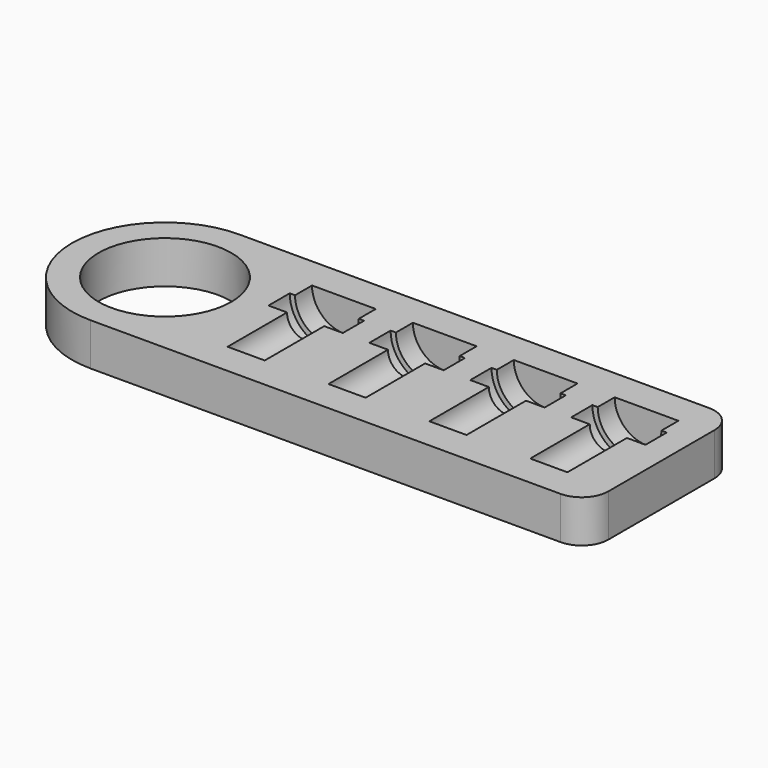
from build123d import *

# Parameters (mm, degrees)
F0_R         = 12.5
F1_DEPTH     = 8
F7_TEXT_SIZE = 5.5555555556
F8_DEPTH     = 1


# Not quite as in the source:
# - Text() gives the source's letters only with a copy of the font that has no kerning and outlines rounded to 1/6400 em; it was checked with that copy


with BuildPart() as f1:
    # F0 (on Top) → F1 (new body)
    with BuildSketch(Plane.XY):
        with BuildLine():
            ThreePointArc((0, 17.5), (5.1256313292, 5.1256313292), (17.5, 0))
            Line((17.5, 0), (106, 0))
            ThreePointArc((106, 0), (109.5355339059, 1.4644660941), (111, 5))
            Line((111, 5), (111, 30))
            ThreePointArc((111, 30), (109.5355339059, 33.5355339059), (106, 35))
            Line((106, 35), (17.5, 35))
            ThreePointArc((17.5, 35), (5.1256313292, 29.8743686708), (0, 17.5))
        make_face()
        with Locations((17.5, 17.5)):
            Circle(F0_R, mode=Mode.SUBTRACT)
    extrude(amount=F1_DEPTH)

    # F2 (on face) → F3 (revolve, cut)
    with BuildSketch(Plane.XY.offset(8)):
        Polygon((42, 20), (42, 6), (45.5, 6), (45.5, 20), (49, 20), (49, 25), (48, 25), (48, 29), (42, 29), (42, 25), align=None)
    revolve(axis=Axis((42, 22.5, 8), (0, 1, 0)), mode=Mode.SUBTRACT)

    # F2 (on face) → F4 (revolve, cut)
    with BuildSketch(Plane.XY.offset(8)):
        Polygon((61, 20), (61, 6), (64.5, 6), (64.5, 20), (68, 20), (68, 25), (67, 25), (67, 29), (61, 29), (61, 25), align=None)
    revolve(axis=Axis((61, 22.5, 8), (0, 1, 0)), mode=Mode.SUBTRACT)

    # F2 (on face) → F5 (revolve, cut)
    with BuildSketch(Plane.XY.offset(8)):
        Polygon((80, 20), (80, 6), (83.5, 6), (83.5, 20), (87, 20), (87, 25), (86, 25), (86, 29), (80, 29), (80, 25), align=None)
    revolve(axis=Axis((80, 13, 8), (0, 1, 0)), mode=Mode.SUBTRACT)

    # F2 (on face) → F6 (revolve, cut)
    with BuildSketch(Plane.XY.offset(8)):
        Polygon((99, 20), (99, 6), (102.5, 6), (102.5, 20), (106, 20), (106, 25), (105, 25), (105, 29), (99, 29), (99, 25), align=None)
    revolve(axis=Axis((99, 13, 8), (0, 1, 0)), mode=Mode.SUBTRACT)

    # F7 (on face) → F8 (cut)
    with BuildSketch(Plane(origin=(0, 0, 0), x_dir=(1, 0, 0), z_dir=(0, 0, -1))):
        with Locations((30, -9)):
            Text('0838, 976', F7_TEXT_SIZE, font='Open Sans', text_align=(TextAlign.LEFT, TextAlign.BOTTOM))
    extrude(amount=-F8_DEPTH, mode=Mode.SUBTRACT)


solid = f1.part
